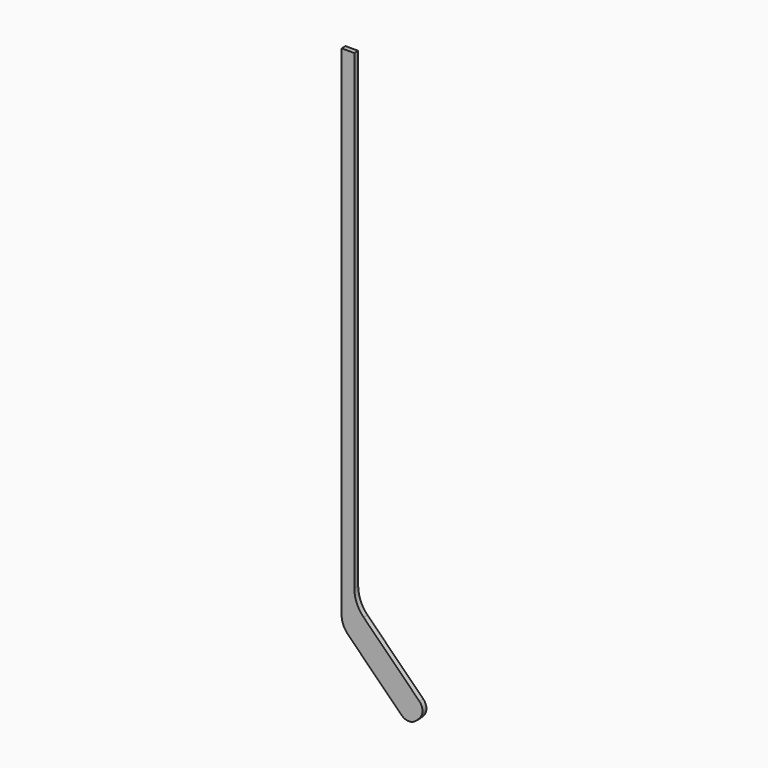
from build123d import *

# Parameters (mm, degrees)
F1_DEPTH = 1.15
F2_R     = 5
F3_R     = 10
F5_R     = 15


with BuildPart() as f1:
    # F0 (on Front) → F1 (new body, symmetric)
    with BuildSketch(Plane.XZ):
        Polygon((0, 240), (0, 0), (31.8198051534, -31.8198051534), (40.3050865276, -23.3345237792), (6, 10.9705627485), (6, 240), align=None)
    extrude(amount=F1_DEPTH, both=True)

    # F2
    f2_edges = [f1.edges().sort_by_distance(p)[0] for p in [
        (31.819805, 0, -31.819805),
        (40.305087, 0, -23.334524),
    ]]
    fillet(f2_edges, radius=F2_R)

    # F3
    f3_edges = [f1.edges().sort_by_distance(p)[0] for p in [
        (0, 0, 0),
    ]]
    fillet(f3_edges, radius=F3_R)

    # F5
    f5_edges = [f1.edges().sort_by_distance(p)[0] for p in [
        (6, 0, 10.970563),
    ]]
    fillet(f5_edges, radius=F5_R)


solid = f1.part
